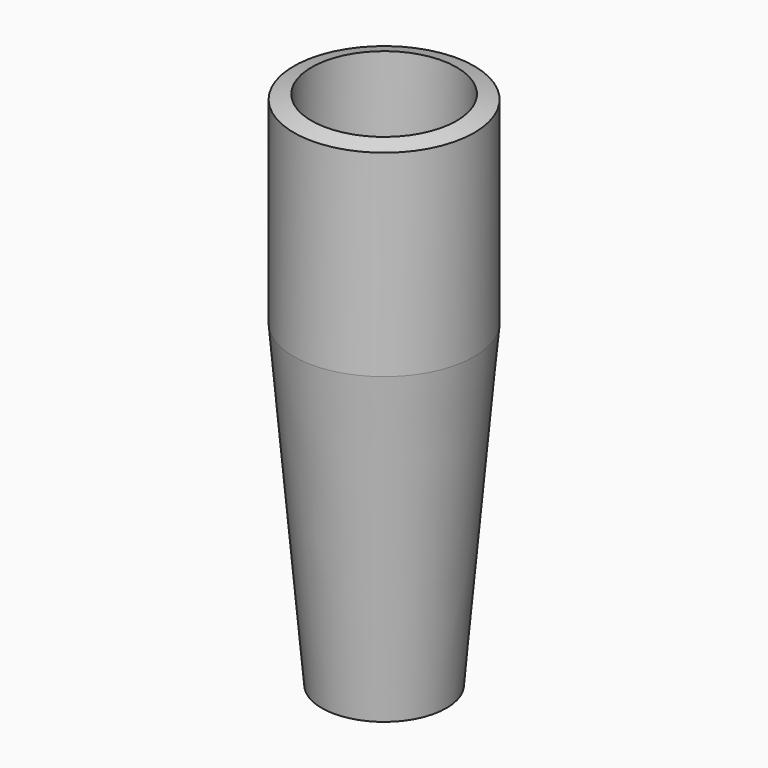
from build123d import *

# Parameters (mm, degrees)
F0_R     = 10.25
F0_R_2   = 5.75
F1_DEPTH = 20
F0_R_3   = 12.75
F2_DEPTH = 35
F3_DEPTH = 40
F5_SIZE2 = 3.9369898587
F5_SIZE  = 45
F7_DEPTH = 25


# Not quite as in the source:
# - a fillet or chamfer that OpenCascade refuses, or shapes differently, is made with other operations: its cross-section is extruded or revolved along the edge and cut away or added


with BuildPart() as f1:
    # F0 (on Top) → F1 (new body)
    with BuildSketch(Plane.XY):
        Circle(F0_R)
        Circle(F0_R_2, mode=Mode.SUBTRACT)
    extrude(amount=F1_DEPTH)

    # F0 (on Top) → F2 (join)
    with BuildSketch(Plane.XY):
        Circle(F0_R_3)
        Circle(F0_R, mode=Mode.SUBTRACT)
    extrude(amount=F2_DEPTH)

    # F3 (add): a face of the model
    f3_faces = [f1.faces().sort_by_distance(p)[0] for p in [
        (-6.1106244584, 0, 0),
    ]]
    extrude(f3_faces, amount=F3_DEPTH)

    # F4: chamfer of 8 x 2.1435935394 on 1 edges, made by hand

    # F4_s1 → F4_t2 (revolve, cut)
    with BuildSketch(Plane.XZ):
        Polygon((12.75, 32.8564064606), (4.75, 35), (12.75, 35), align=None)
    revolve(axis=Axis((0, 0, 35), (0, 0, 1)), mode=Mode.SUBTRACT)

    # F5
    f5_edges = [f1.edges().sort_by_distance(p)[0] for p in [
        (-12.75, 0, -40),
    ]]
    f5_side = f1.faces().sort_by_distance((-12.75, 0, -3.571797))[0]
    chamfer(f5_edges, length=F5_SIZE, length2=F5_SIZE2, reference=f5_side)

    # F6 (on Right) → F7 (cut)
    with BuildSketch(Plane.YZ):
        with BuildLine():
            ThreePointArc((0, -11.2528902143), (-1.5, -12.7528902143), (0, -14.2528902143))
            Line((0, -14.2528902143), (0, -11.2528902143))
        make_face()
        with BuildLine():
            Line((0, -11.2528902143), (0, -14.2528902143))
            ThreePointArc((0, -14.2528902143), (1.0606601718, -13.8135503861), (1.5, -12.7528902143))
            ThreePointArc((1.5, -12.7528902143), (1.0606601718, -11.6922300425), (0, -11.2528902143))
        make_face()
    extrude(amount=-F7_DEPTH, mode=Mode.SUBTRACT)


solid = f1.part
